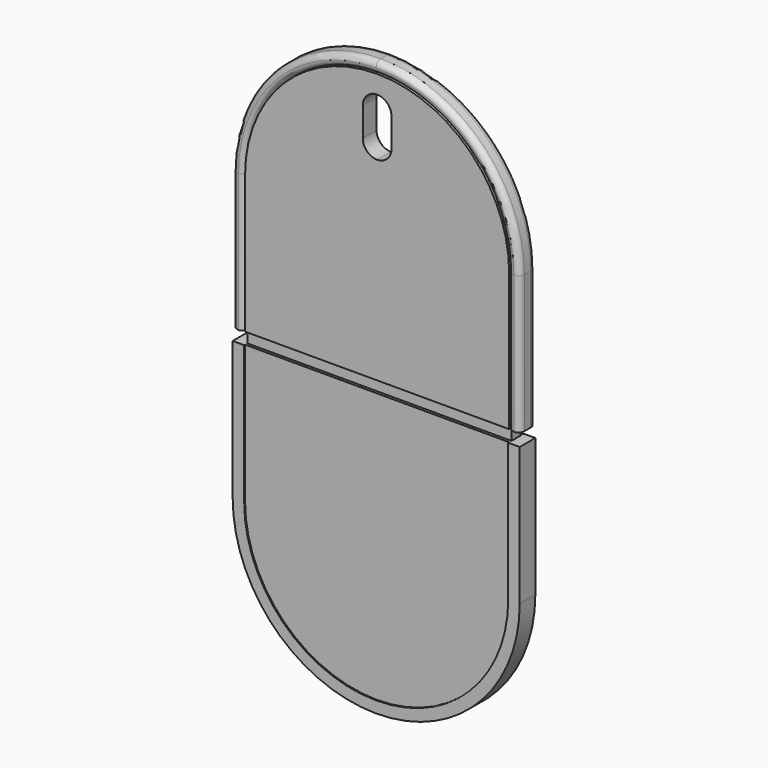
from build123d import *

# Parameters (mm, degrees)
F1_DEPTH      = 0.85
F1_DEPTH_BACK = 0.85
F2_R          = 12.49999
F2_2_R        = 12.49999
F0_W          = 23
F0_H          = 1
F3_DEPTH      = 0.5
F3_DEPTH_BACK = 0.5
F0_W_2        = 2.5
F0_H_2        = 5
F4_DEPTH      = 0.75
F4_DEPTH_BACK = 0.75
F5_T1_DEPTH   = 1.5
F6_R          = 0.49999


# Not quite as in the source:
# - a fillet or chamfer that OpenCascade refuses, or shapes differently, is made with other operations: its cross-section is extruded or revolved along the edge and cut away or added
# - a fillet or chamfer is up to 0.001 mm smaller than in the source, because OpenCascade refuses the exact size
# - a feature names something its author has since deleted; it is built from what else it names


with BuildPart() as f1:
    # F0 (on Front) → F1 (new body, two sides)
    with BuildSketch(Plane.XZ) as f1_sk:
        with BuildLine():
            Line((12.5, 0.5), (12.5, 25))
            Line((12.5, 25), (-12.5, 25))
            Line((-12.5, 25), (-12.5, 0.5))
            Line((-12.5, 0.5), (-11.5, 0.5))
            Line((-11.5, 0.5), (-11.5, 12.5))
            ThreePointArc((-11.5, 12.5), (-8.1317279836, 20.6317279836), (0, 24))
            ThreePointArc((0, 24), (8.1317279836, 20.6317279836), (11.5, 12.5))
            Line((11.5, 12.5), (11.5, 0.5))
            Line((11.5, 0.5), (12.5, 0.5))
        make_face()
    extrude(amount=F1_DEPTH)
    extrude(f1_sk.sketch, amount=-F1_DEPTH_BACK)

    # F2 (radius 12.5 in the source; OpenCascade refuses exactly that, so slightly less here)
    f2_edges = [f1.edges().sort_by_distance(p)[0] for p in [
        (12.5, 0, 25),
        (-12.5, 0, 25),
    ]]
    fillet(f2_edges, radius=F2_R)

    # F6 (radius 0.5 in the source; OpenCascade refuses exactly that, so slightly less here)
    f6_edges = [f1.edges().sort_by_distance(p)[0] for p in [
        (8.838838, -0.85, 21.338838),
        (12.5, -0.85, 6.500005),
        (12.5, 0.85, 6.500005),
        (8.838838, 0.85, 21.338838),
        (-12.5, -0.85, 6.500005),
        (-12.5, 0.85, 6.500005),
        (-11.5, -0.85, 6.5),
        (0, -0.85, 24),
        (11.5, 0.85, 6.5),
        (0, 0.85, 24),
        (-11.5, 0.85, 6.5),
        (11.5, -0.85, 6.5),
        (0, -0.85, 25),
        (-8.838838, -0.85, 21.338838),
        (0, 0.85, 25),
        (-8.838838, 0.85, 21.338838),
    ]]
    fillet(f6_edges, radius=F6_R)


with BuildPart() as f1b:
    # F0 (on Front) → F1, piece 2 (new body, two sides)
    with BuildSketch(Plane.XZ) as f1_2_sk:
        with BuildLine():
            Line((12.5, -25), (12.5, -0.5))
            Line((12.5, -0.5), (11.5, -0.5))
            Line((11.5, -0.5), (11.5, -12.5))
            ThreePointArc((11.5, -12.5), (8.1317279836, -20.6317279836), (0, -24))
            ThreePointArc((0, -24), (-8.1317279836, -20.6317279836), (-11.5, -12.5))
            Line((-11.5, -12.5), (-11.5, -0.5))
            Line((-11.5, -0.5), (-12.5, -0.5))
            Line((-12.5, -0.5), (-12.5, -25))
            Line((-12.5, -25), (12.5, -25))
        make_face()
    extrude(amount=F1_DEPTH)
    extrude(f1_2_sk.sketch, amount=-F1_DEPTH_BACK)

    # F2#2 (radius 12.5 in the source; OpenCascade refuses exactly that, so slightly less here)
    f2_2_edges = [f1b.edges().sort_by_distance(p)[0] for p in [
        (12.5, 0, -25),
        (-12.5, 0, -25),
    ]]
    fillet(f2_2_edges, radius=F2_2_R)


with BuildPart() as f3:
    # F0 (on Front) → F3 (new body, two sides)
    with BuildSketch(Plane.XZ) as f3_sk:
        Rectangle(F0_W, F0_H)
    extrude(amount=F3_DEPTH)
    extrude(f3_sk.sketch, amount=-F3_DEPTH_BACK)


with BuildPart() as f4:
    # F0 (on Front) → F4 (new body, two sides)
    with BuildSketch(Plane.XZ) as f4_sk:
        with BuildLine():
            Line((-11.5, 0.5), (11.5, 0.5))
            Line((11.5, 0.5), (11.5, 12.5))
            ThreePointArc((11.5, 12.5), (8.1317279836, 20.6317279836), (0, 24))
            ThreePointArc((0, 24), (-8.1317279836, 20.6317279836), (-11.5, 12.5))
            Line((-11.5, 12.5), (-11.5, 0.5))
        make_face()
        with Locations((0, 19.9144259095)):
            Rectangle(F0_W_2, F0_H_2, mode=Mode.SUBTRACT)
    extrude(amount=F4_DEPTH)
    extrude(f4_sk.sketch, amount=-F4_DEPTH_BACK)

    # F5: fillet of radius 1.25 on 4 edges, made by hand

    # F5_s2 → F5_t1 (join)
    with BuildSketch(Plane.XZ.offset(-0.75)):
        with BuildLine():
            ThreePointArc((0, 22.4144259095), (-0.8838834765, 22.048309386), (-1.25, 21.1644259095))
            Line((-1.25, 21.1644259095), (-1.25, 22.4144259095))
            Line((-1.25, 22.4144259095), (0, 22.4144259095))
        make_face()
        with BuildLine():
            ThreePointArc((0, 22.4144259095), (0.8838834765, 22.048309386), (1.25, 21.1644259095))
            Line((1.25, 21.1644259095), (1.25, 22.4144259095))
            Line((1.25, 22.4144259095), (0, 22.4144259095))
        make_face()
        with BuildLine():
            ThreePointArc((-1.25, 18.6644259095), (-0.8838834765, 17.780542433), (0, 17.4144259095))
            Line((0, 17.4144259095), (-1.25, 17.4144259095))
            Line((-1.25, 17.4144259095), (-1.25, 18.6644259095))
        make_face()
        with BuildLine():
            ThreePointArc((0, 17.4144259095), (0.8838834765, 17.780542433), (1.25, 18.6644259095))
            Line((1.25, 18.6644259095), (1.25, 17.4144259095))
            Line((1.25, 17.4144259095), (0, 17.4144259095))
        make_face()
    extrude(amount=F5_T1_DEPTH)


with BuildPart() as f4b:
    # F0 (on Front) → F4, piece 2 (new body, two sides)
    with BuildSketch(Plane.XZ) as f4_2_sk:
        with BuildLine():
            Line((11.5, -12.5), (11.5, -0.5))
            Line((11.5, -0.5), (-11.5, -0.5))
            Line((-11.5, -0.5), (-11.5, -12.5))
            ThreePointArc((-11.5, -12.5), (-8.1317279836, -20.6317279836), (0, -24))
            ThreePointArc((0, -24), (8.1317279836, -20.6317279836), (11.5, -12.5))
        make_face()
    extrude(amount=F4_DEPTH)
    extrude(f4_2_sk.sketch, amount=-F4_DEPTH_BACK)


solid = Compound([f1.part, f1b.part, f3.part, f4.part, f4b.part])
